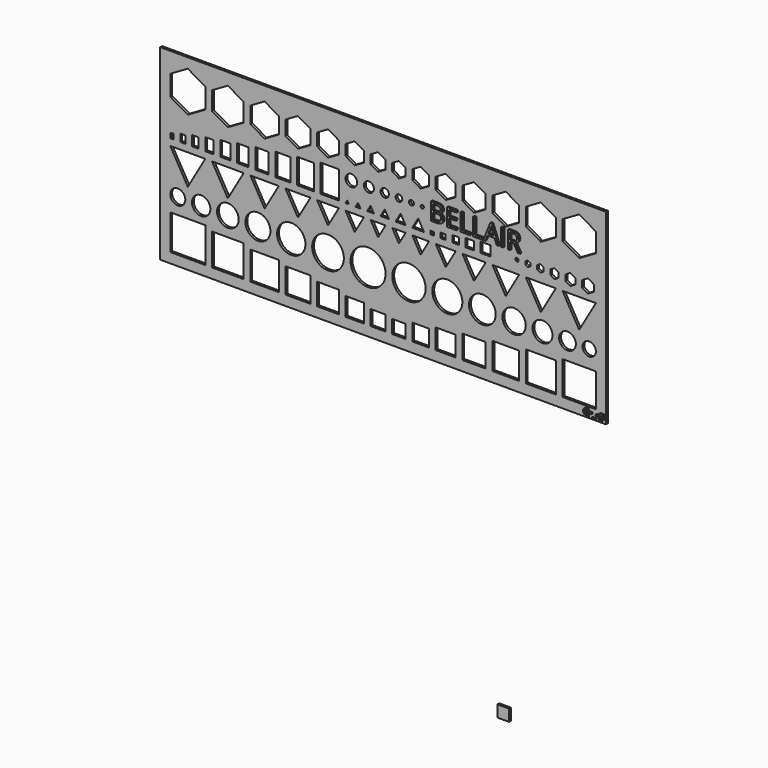
from build123d import *

# Parameters (mm, degrees)
F0_W         = 7
F0_H         = 7
F1_DEPTH     = 1.4
F0_W_2       = 267
F0_H_2       = 112.1280236695
F0_W_3       = 21
F0_H_3       = 21
F0_R         = 4.5
F0_R_2       = 5.5
F0_W_4       = 19
F0_H_4       = 19
F0_W_5       = 17
F0_H_5       = 17
F0_R_3       = 6.5
F0_R_4       = 7.5
F0_W_6       = 15
F0_H_6       = 15
F0_R_5       = 8.5
F0_W_7       = 13
F0_H_7       = 13
F0_W_8       = 11
F0_H_8       = 11
F0_W_9       = 9
F0_H_9       = 9
F0_R_6       = 9.5
F0_R_7       = 10.5
F0_W_10      = 2
F0_H_10      = 3
F0_W_11      = 3
F0_H_11      = 4.5
F0_W_12      = 4
F0_H_12      = 6
F0_W_13      = 5
F0_H_13      = 7.5
F0_W_14      = 6
F0_H_14      = 10.5
F0_W_15      = 8
F0_H_15      = 12
F0_H_16      = 13.5
F0_W_16      = 10
F0_H_17      = 16.5
F0_R_8       = 3
F0_H_18      = 8
F0_H_19      = 10
F0_R_9       = 10
F0_W_17      = 12
F0_W_18      = 14
F0_H_20      = 14
F0_R_10      = 9
F0_R_11      = 8
F0_W_19      = 16
F0_H_21      = 16
F0_W_20      = 18
F0_H_22      = 18
F0_R_12      = 7
F0_R_13      = 6
F0_W_21      = 20
F0_H_23      = 20
F0_R_14      = 5
F0_R_15      = 4
F0_H_24      = 2
F0_H_25      = 4
F0_H_26      = 5
F0_R_16      = 2.5
F0_R_17      = 2
F0_R_18      = 1.5
F0_R_19      = 1
F2_TEXT_SIZE = 14.5815519823
F3_DEPTH     = 1
F4_TEXT_SIZE = 5.6002633859
F5_DEPTH     = 1


# Not quite as in the source:
# - Text() gives the source's letters only with a copy of the font that has no kerning and outlines rounded to 1/6400 em; it was checked with that copy


with BuildPart() as f1:
    # F0 (on Front) → F1 (new body)
    with BuildSketch(Plane.XZ):
        with Locations((66.5000000737, -178.3107280108)):
            Rectangle(F0_W, F0_H)
    extrude(amount=F1_DEPTH)


with BuildPart() as f1b:
    # F0 (on Front) → F1, piece 2 (new body)
    with BuildSketch(Plane.XZ):
        with Locations((-5.5, 50.0640118348)):
            Rectangle(F0_W_2, F0_H_2)
        with Locations((-122.5, 10.5)):
            Rectangle(F0_W_3, F0_H_3, mode=Mode.SUBTRACT)
        with Locations((-128.5, 30.5)):
            Circle(F0_R, mode=Mode.SUBTRACT)
        with Locations((-114.5, 30.5)):
            Circle(F0_R_2, mode=Mode.SUBTRACT)
        with Locations((-98.5, 9.5)):
            Rectangle(F0_W_4, F0_H_4, mode=Mode.SUBTRACT)
        with Locations((-76.5, 8.5)):
            Rectangle(F0_W_5, F0_H_5, mode=Mode.SUBTRACT)
        with Locations((-98.5, 30.4999999999)):
            Circle(F0_R_3, mode=Mode.SUBTRACT)
        with Locations((-80.5, 30.4999999999)):
            Circle(F0_R_4, mode=Mode.SUBTRACT)
        with Locations((-56.5, 7.5000000003)):
            Rectangle(F0_W_6, F0_H_6, mode=Mode.SUBTRACT)
        with Locations((-60.5, 30.5)):
            Circle(F0_R_5, mode=Mode.SUBTRACT)
        with Locations((-38.5, 6.5)):
            Rectangle(F0_W_7, F0_H_7, mode=Mode.SUBTRACT)
        with Locations((-22.5, 5.5)):
            Rectangle(F0_W_8, F0_H_8, mode=Mode.SUBTRACT)
        with Locations((-8.5, 4.5)):
            Rectangle(F0_W_9, F0_H_9, mode=Mode.SUBTRACT)
        with Locations((-38.5, 30.5)):
            Circle(F0_R_6, mode=Mode.SUBTRACT)
        with Locations((-14.5, 30.5)):
            Circle(F0_R_7, mode=Mode.SUBTRACT)
        Polygon((-122.5000000002, 37.8115810376), (-133.0000000002, 55.9981145171), (-112.0000000002, 55.9981145171), align=None, mode=Mode.SUBTRACT)
        with Locations((-131.9999999263, 61.4981145171)):
            Rectangle(F0_W_10, F0_H_10, mode=Mode.SUBTRACT)
        with Locations((-125.4999999263, 62.2481145171)):
            Rectangle(F0_W_11, F0_H_11, mode=Mode.SUBTRACT)
        with Locations((-117.9999999263, 62.9981145171)):
            Rectangle(F0_W_12, F0_H_12, mode=Mode.SUBTRACT)
        with Locations((-109.4999999263, 63.7481145171)):
            Rectangle(F0_W_13, F0_H_13, mode=Mode.SUBTRACT)
        Polygon((-98.5000000002, 39.5436318452), (-108.0000000002, 55.9981145171), (-89.0000000002, 55.9981145171), align=None, mode=Mode.SUBTRACT)
        Polygon((-76.5000000002, 41.2756826531), (-85.0000000002, 55.9981145174), (-68.0000000002, 55.9981145174), align=None, mode=Mode.SUBTRACT)
        with Locations((-99.9999999263, 64.4981145171)):
            Rectangle(F0_W_14, F0_H_9, mode=Mode.SUBTRACT)
        with Locations((-89.4999999263, 65.2481145171)):
            Rectangle(F0_W, F0_H_14, mode=Mode.SUBTRACT)
        with Locations((-77.9999999263, 65.9981145171)):
            Rectangle(F0_W_15, F0_H_15, mode=Mode.SUBTRACT)
        Polygon((-122.5, 100.1280236695), (-112, 94.065845843), (-112, 81.94149019), (-122.5, 75.8793123636), (-133, 81.94149019), (-133, 94.065845843), align=None, mode=Mode.SUBTRACT)
        Polygon((-98.5, 77.0340129019), (-108, 82.5188404592), (-108, 93.4884955738), (-98.5, 98.9733231311), (-89, 93.4884955738), (-89, 82.5188404592), align=None, mode=Mode.SUBTRACT)
        Polygon((-76.5, 78.1887134403), (-85, 83.0961907284), (-85, 92.9111453047), (-76.5, 97.8186225928), (-68, 92.9111453047), (-68, 83.0961907284), align=None, mode=Mode.SUBTRACT)
        Polygon((-56.5000000002, 43.0077334606), (-64.0000000002, 55.9981145174), (-49.0000000002, 55.9981145174), align=None, mode=Mode.SUBTRACT)
        with Locations((-65.4999999263, 66.7481145171)):
            Rectangle(F0_W_9, F0_H_16, mode=Mode.SUBTRACT)
        with Locations((-51.9999999263, 67.4981145171)):
            Rectangle(F0_W_16, F0_H_6, mode=Mode.SUBTRACT)
        Polygon((-38.5000000002, 44.7397842682), (-45.0000000002, 55.9981145174), (-32.0000000002, 55.9981145174), align=None, mode=Mode.SUBTRACT)
        Polygon((-22.5000000002, 46.4718350758), (-28.0000000002, 55.9981145174), (-17.0000000002, 55.9981145174), align=None, mode=Mode.SUBTRACT)
        Polygon((-8.5000000004, 48.2038858834), (-13.0000000002, 55.9981145176), (-4.0000000002, 55.9981145174), align=None, mode=Mode.SUBTRACT)
        Polygon((-26.9999999263, 61.7301653326), (-25.9999999263, 59.9981145251), (-27.9999999263, 59.9981145251), align=None, mode=Mode.SUBTRACT)
        with Locations((-37.4999999263, 68.2481145171)):
            Rectangle(F0_W_8, F0_H_17, mode=Mode.SUBTRACT)
        Polygon((-20.4999999276, 62.5961907282), (-18.9999999263, 59.9981145176), (-21.9999999263, 59.998114516), align=None, mode=Mode.SUBTRACT)
        Polygon((-12.9999999263, 63.4622161402), (-10.9999999263, 59.9981145251), (-14.9999999263, 59.9981145251), align=None, mode=Mode.SUBTRACT)
        Polygon((-56.5, 96.6639220544), (-49, 92.3337950355), (-49, 83.6735409976), (-56.5, 79.3434139787), (-64, 83.6735409976), (-64, 92.3337950355), align=None, mode=Mode.SUBTRACT)
        with BuildLine():
            ThreePointArc((-21, 72.9981145171), (-24.5, 69.4981145171), (-28, 72.9981145171))
            ThreePointArc((-28, 72.9981145171), (-24.5, 76.4981145171), (-21, 72.9981145171))
        make_face(mode=Mode.SUBTRACT)
        Polygon((-38.5, 95.509221516), (-32, 91.7564447663), (-32, 84.2508912668), (-38.5, 80.4981145171), (-45, 84.2508912668), (-45, 91.7564447663), align=None, mode=Mode.SUBTRACT)
        Polygon((-22.5, 81.6528150555), (-28, 84.828241536), (-28, 91.1790944971), (-22.5, 94.3545209776), (-17, 91.1790944971), (-17, 84.828241536), align=None, mode=Mode.SUBTRACT)
        with Locations((-14, 72.9981145171)):
            Circle(F0_R_8, mode=Mode.SUBTRACT)
        Polygon((-8.5, 82.8075155938), (-13, 85.4055918052), (-13, 90.6017442279), (-8.5, 93.1998204392), (-4, 90.6017442279), (-4, 85.4055918052), align=None, mode=Mode.SUBTRACT)
        with Locations((4, 4)):
            Rectangle(F0_W_15, F0_H_18, mode=Mode.SUBTRACT)
        with Locations((17, 5)):
            Rectangle(F0_W_16, F0_H_19, mode=Mode.SUBTRACT)
        with Locations((10, 30.5)):
            Circle(F0_R_9, mode=Mode.SUBTRACT)
        with Locations((32, 6)):
            Rectangle(F0_W_17, F0_H_15, mode=Mode.SUBTRACT)
        with Locations((49, 7)):
            Rectangle(F0_W_18, F0_H_20, mode=Mode.SUBTRACT)
        with Locations((33, 30.5)):
            Circle(F0_R_10, mode=Mode.SUBTRACT)
        with Locations((54, 30.5)):
            Circle(F0_R_11, mode=Mode.SUBTRACT)
        with Locations((68, 8)):
            Rectangle(F0_W_19, F0_H_21, mode=Mode.SUBTRACT)
        with Locations((89, 9)):
            Rectangle(F0_W_20, F0_H_22, mode=Mode.SUBTRACT)
        with Locations((73, 30.5)):
            Circle(F0_R_12, mode=Mode.SUBTRACT)
        with Locations((90, 30.5)):
            Circle(F0_R_13, mode=Mode.SUBTRACT)
        with Locations((112, 10)):
            Rectangle(F0_W_21, F0_H_23, mode=Mode.SUBTRACT)
        with Locations((105, 30.5)):
            Circle(F0_R_14, mode=Mode.SUBTRACT)
        with Locations((118, 30.5)):
            Circle(F0_R_15, mode=Mode.SUBTRACT)
        Polygon((17, 47.3378604792), (12, 55.9981145171), (22, 55.9981145171), align=None, mode=Mode.SUBTRACT)
        Polygon((3.9999999999, 49.0699112869), (-2e-10, 55.9981145174), (8, 55.9981145174), align=None, mode=Mode.SUBTRACT)
        Polygon((-4.4999999263, 64.3282415484), (-1.9999999263, 59.9981145294), (-6.9999999263, 59.9981145294), align=None, mode=Mode.SUBTRACT)
        Polygon((5.0000000737, 65.1942669514), (8.0000000737, 59.9981145287), (2.0000000737, 59.9981145287), align=None, mode=Mode.SUBTRACT)
        with Locations((24.0000000737, 60.9981145171)):
            Rectangle(F0_W_10, F0_H_24, mode=Mode.SUBTRACT)
        Polygon((15.5000000737, 66.0602923559), (19.0000000737, 59.9981145294), (12.0000000737, 59.9981145294), align=None, mode=Mode.SUBTRACT)
        Polygon((32, 45.6058096717), (26, 55.9981145171), (38, 55.9981145171), align=None, mode=Mode.SUBTRACT)
        Polygon((49, 43.8737588641), (42, 55.9981145171), (56, 55.9981145171), align=None, mode=Mode.SUBTRACT)
        with Locations((30.5000000737, 61.4981145171)):
            Rectangle(F0_W_11, F0_H_10, mode=Mode.SUBTRACT)
        with Locations((38.0000000737, 61.9981145171)):
            Rectangle(F0_W_12, F0_H_25, mode=Mode.SUBTRACT)
        with Locations((46.5000000737, 62.4981145171)):
            Rectangle(F0_W_13, F0_H_26, mode=Mode.SUBTRACT)
        with Locations((56.0000000737, 62.9981145171)):
            Rectangle(F0_W_14, F0_H_12, mode=Mode.SUBTRACT)
        with Locations((-4.5, 72.9981145171)):
            Circle(F0_R_16, mode=Mode.SUBTRACT)
        with Locations((4, 72.9981145171)):
            Circle(F0_R_17, mode=Mode.SUBTRACT)
        Polygon((4, 83.384865863), (0, 85.6942669398), (0, 90.3130690933), (4, 92.6224701701), (8, 90.3130690933), (8, 85.6942669398), align=None, mode=Mode.SUBTRACT)
        with Locations((11.5, 72.9981145171)):
            Circle(F0_R_18, mode=Mode.SUBTRACT)
        with Locations((18, 72.9981145171)):
            Circle(F0_R_19, mode=Mode.SUBTRACT)
        Polygon((17, 93.7771707084), (22, 90.8904193625), (22, 85.1169166706), (17, 82.2301653246), (12, 85.1169166706), (12, 90.8904193625), align=None, mode=Mode.SUBTRACT)
        Polygon((32, 81.0754647863), (26, 84.5395664014), (26, 91.4677696317), (32, 94.9318712468), (38, 91.4677696317), (38, 84.5395664014), align=None, mode=Mode.SUBTRACT)
        Polygon((49, 79.9207642479), (42, 83.9622161322), (42, 92.0451199009), (49, 96.0865717852), (56, 92.0451199009), (56, 83.9622161322), align=None, mode=Mode.SUBTRACT)
        Polygon((68, 42.1417080565), (60, 55.9981145171), (76, 55.9981145171), align=None, mode=Mode.SUBTRACT)
        Polygon((89, 40.409657249), (80, 55.9981145171), (98, 55.9981145171), align=None, mode=Mode.SUBTRACT)
        Polygon((74.7341739481, 64.6528143443), (75.7348142498, 64.0765745332), (75.7360960856, 62.9218747063), (74.7367376196, 62.3434146905), (73.7360973179, 62.9196545016), (73.7348154821, 64.0743543285), align=None, mode=Mode.SUBTRACT)
        Polygon((81.2335370352, 65.2301642578), (82.7344974878, 64.3658045411), (82.7364202415, 62.6337548008), (81.2373825426, 61.7660647771), (79.73642209, 62.6304244937), (79.7344993363, 64.362474234), align=None, mode=Mode.SUBTRACT)
        Polygon((88.7380280817, 61.1887148636), (86.7367474783, 62.3411944858), (86.7341838067, 64.6505941396), (88.7329007386, 65.8075141712), (90.734181342, 64.655034549), (90.7367450136, 62.3456348952), align=None, mode=Mode.SUBTRACT)
        Polygon((112, 38.6776064417), (102, 55.9981145174), (122, 55.9981145174), align=None, mode=Mode.SUBTRACT)
        Polygon((97.2322650581, 66.3848640846), (99.7338658124, 64.9442645569), (99.7370704019, 62.0575149897), (97.238674237, 60.6113649502), (94.7370734827, 62.0519644779), (94.7338688932, 64.9387140451), align=None, mode=Mode.SUBTRACT)
        Polygon((106.7316299937, 66.9622139981), (109.7335508989, 65.2334945648), (109.7373964063, 61.7693950841), (106.7393210085, 60.0340150367), (103.7374001033, 61.76273447), (103.7335545959, 65.2268339507), align=None, mode=Mode.SUBTRACT)
        Polygon((117.2309955456, 67.5395639115), (120.7332366016, 65.5227245727), (120.7377230269, 61.4812751786), (117.2399683961, 59.4566651233), (113.73772734, 61.4735044621), (113.7332409148, 65.5149538562), align=None, mode=Mode.SUBTRACT)
        Polygon((68, 78.7660637095), (60, 83.384865863), (60, 92.6224701701), (68, 97.2412723236), (76, 92.6224701701), (76, 83.384865863), align=None, mode=Mode.SUBTRACT)
        Polygon((89, 77.6113631711), (80, 82.8075155938), (80, 93.1998204392), (89, 98.395972862), (98, 93.1998204392), (98, 82.8075155938), align=None, mode=Mode.SUBTRACT)
        Polygon((112, 76.4566626327), (102, 82.2301653246), (102, 93.7771707084), (112, 99.5506734003), (122, 93.7771707084), (122, 82.2301653246), align=None, mode=Mode.SUBTRACT)
    extrude(amount=F1_DEPTH)

    # F2 (on face) → F3 (join)
    with BuildSketch(Plane.XZ.offset(1.4)):
        with Locations((22.6940829307, 67.9160133004)):
            Text('BELLAIR', F2_TEXT_SIZE, font='Open Sans', text_align=(TextAlign.LEFT, TextAlign.BOTTOM))
    extrude(amount=F3_DEPTH)

    # F4 (on face) → F5 (join)
    with BuildSketch(Plane.XZ.offset(1.4)):
        with Locations((114.8945086359, -4.0321896378)):
            Text('q-_-p', F4_TEXT_SIZE, font='Open Sans', font_style=FontStyle.BOLD, text_align=(TextAlign.LEFT, TextAlign.BOTTOM))
    extrude(amount=F5_DEPTH)


solid = Compound([f1.part, f1b.part])
